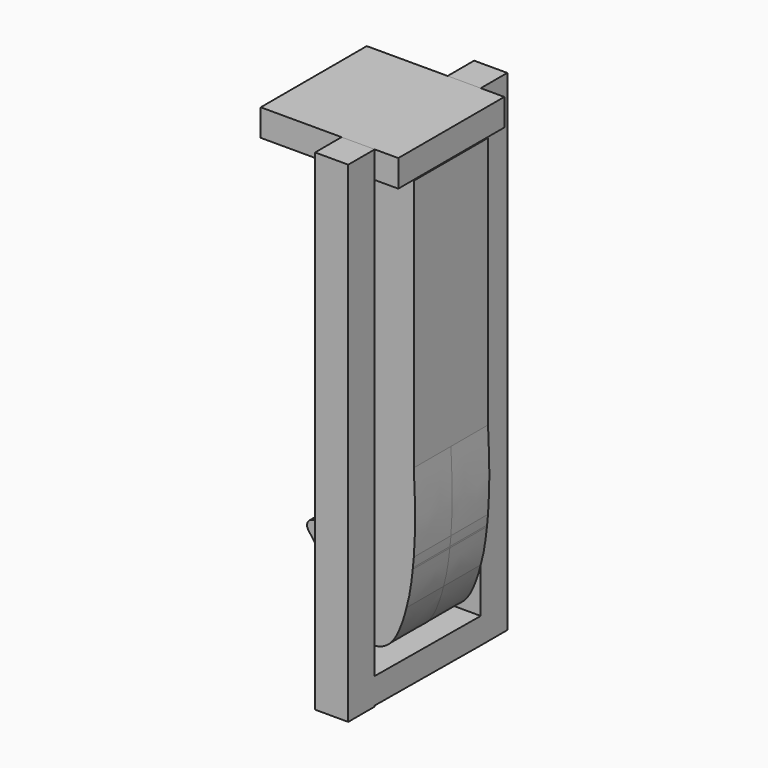
from build123d import *

# Parameters (mm, degrees)
F1_DEPTH = 8.89
F2_R     = 1.27
F3_R     = 1.27
F4_W     = 26.3627418317
F4_H     = 5.1619373262
F5_DEPTH = 12.7
F7_DEPTH = 6.35


with BuildPart() as f1:
    # F0 (on Front) → F1 (new body, symmetric)
    with BuildSketch(Plane.XZ):
        with BuildLine():
            add(Edge.make_bspline(
                [(4.2661379753, -33.616950048), (4.3349248687, -32.99222106), (4.3945578489, -32.36840068), (4.445, -31.75)],
                knots=[0.4799922653, 0.4799922653, 0.4799922653, 0.4799922653, 0.5123717025, 0.5123717025, 0.5123717025, 0.5123717025], degree=3))
            Line((4.445, -31.75), (-4.445, -31.75))
            Line((-4.445, -31.75), (-17.2371771187, -31.75))
            Line((-17.2371771187, -31.75), (-4.445, -49.3149235845))
            add(Edge.make_bspline(
                [(-4.445, -49.3149235845), (-2.8737867331, -49.1791167069), (-1.3025734662, -49.0433098293), (0, -47.6557277143)],
                knots=[0, 0, 0, 0, 0.1787943452, 0.1787943452, 0.1787943452, 0.1787943452], degree=3))
            add(Edge.make_bspline(
                [(0, -47.6557277143), (1.1546532493, -45.3808190167), (2.3218615323, -43.1096212641), (3.0350551164, -40.743494961)],
                knots=[0, 0, 0, 0, 0.5053639981, 0.5053639981, 0.5053639981, 0.5053639981], degree=3))
            add(Edge.make_bspline(
                [(3.0350551164, -40.743494961), (3.5641678247, -38.6195342287), (3.9647615791, -36.2559041312), (4.2348473132, -33.8956672077)],
                knots=[0.3528810834, 0.3528810834, 0.3528810834, 0.3528810834, 0.4751777864, 0.4751777864, 0.4751777864, 0.4751777864], degree=3))
            add(Edge.make_bspline(
                [(4.2348473132, -33.8956672077), (4.2452843652, -33.8027605788), (4.2557060854, -33.7098530506), (4.2661379753, -33.616950048)],
                knots=[0.9808831842, 0.9808831842, 0.9808831842, 0.9808831842, 1, 1, 1, 1], degree=3))
        make_face()
        with BuildLine():
            Line((-4.445, -31.75), (4.445, -31.75))
            Line((4.445, -31.75), (4.445, -16.6841130704))
            add(Edge.make_bspline(
                [(4.445, -16.6841130704), (4.390455432, -14.8693285963), (4.417727716, -13.6566404294), (4.445, -12.4439522624)],
                knots=[0.830976746, 0.830976746, 0.830976746, 0.830976746, 1, 1, 1, 1], degree=3))
            Line((4.445, -12.4439522624), (4.445, 31.75))
            Line((4.445, 31.75), (-4.445, 31.75))
            Line((-4.445, 31.75), (-4.445, -31.75))
        make_face()
        with BuildLine():
            Line((4.445, -16.6841130704), (4.445, -31.75))
            add(Edge.make_bspline(
                [(4.445, -31.75), (4.9413373419, -25.665101898), (4.5478152875, -20.1049411089), (4.445, -16.6841130704)],
                knots=[0.5123717025, 0.5123717025, 0.5123717025, 0.5123717025, 0.830976746, 0.830976746, 0.830976746, 0.830976746], degree=3))
        make_face()
        with BuildLine():
            add(Edge.make_bspline(
                [(4.445, -16.6841130704), (4.390455432, -14.8693285963), (4.417727716, -13.6566404294), (4.445, -12.4439522624)],
                knots=[0.830976746, 0.830976746, 0.830976746, 0.830976746, 1, 1, 1, 1], degree=3))
            Line((4.445, -16.6841130704), (4.445, -12.4439522624))
        make_face()
        with BuildLine():
            add(Edge.make_bspline(
                [(4.2348473132, -33.8956672077), (4.2454798326, -33.802751286), (4.2559100938, -33.709840623), (4.2661379753, -33.616950048)],
                knots=[0.4751777864, 0.4751777864, 0.4751777864, 0.4751777864, 0.4799922653, 0.4799922653, 0.4799922653, 0.4799922653], degree=3))
            add(Edge.make_bspline(
                [(4.2348473132, -33.8956672077), (4.2452843652, -33.8027605788), (4.2557060854, -33.7098530506), (4.2661379753, -33.616950048)],
                knots=[0.9808831842, 0.9808831842, 0.9808831842, 0.9808831842, 1, 1, 1, 1], degree=3))
        make_face()
        with BuildLine():
            add(Edge.make_bspline(
                [(3.0350551164, -40.743494961), (3.7061302896, -38.5171027806), (3.9752319818, -36.2066631893), (4.2348473132, -33.8956672077)],
                knots=[0.5053639981, 0.5053639981, 0.5053639981, 0.5053639981, 0.9808831842, 0.9808831842, 0.9808831842, 0.9808831842], degree=3))
            add(Edge.make_bspline(
                [(3.0350551164, -40.743494961), (3.5641678247, -38.6195342287), (3.9647615791, -36.2559041312), (4.2348473132, -33.8956672077)],
                knots=[0.3528810834, 0.3528810834, 0.3528810834, 0.3528810834, 0.4751777864, 0.4751777864, 0.4751777864, 0.4751777864], degree=3))
        make_face()
        with BuildLine():
            add(Edge.make_bspline(
                [(0, -47.6557277143), (1.2682770572, -46.3046802631), (2.2818745053, -43.7669075859), (3.0350551164, -40.743494961)],
                knots=[0.1787943452, 0.1787943452, 0.1787943452, 0.1787943452, 0.3528810834, 0.3528810834, 0.3528810834, 0.3528810834], degree=3))
            add(Edge.make_bspline(
                [(0, -47.6557277143), (1.1546532493, -45.3808190167), (2.3218615323, -43.1096212641), (3.0350551164, -40.743494961)],
                knots=[0, 0, 0, 0, 0.5053639981, 0.5053639981, 0.5053639981, 0.5053639981], degree=3))
        make_face()
    extrude(amount=F1_DEPTH, both=True)

    # F2
    f2_edges = [f1.edges().sort_by_distance(p)[0] for p in [
        (-17.237177, 0, -31.75),
    ]]
    fillet(f2_edges, radius=F2_R)

    # F3
    f3_edges = [f1.edges().sort_by_distance(p)[0] for p in [
        (-4.445, 4.445, -49.314924),
        (-4.445, -4.445, -49.314924),
    ]]
    fillet(f3_edges, radius=F3_R)


with BuildPart() as f5:
    # F4 (on Front) → F5 (new body, symmetric)
    with BuildSketch(Plane.XZ):
        with Locations((-8.6646776181, 34.5665309578)):
            Rectangle(F4_W, F4_H)
    extrude(amount=F5_DEPTH, both=True)


with BuildPart() as f7:
    # F6 (on Right) → F7 (new body)
    with BuildSketch(Plane.YZ):
        Polygon((19.05, 37.1474996209), (12.7, 37.1474996209), (12.7, -51.8958903849), (12.7, -56.8734705448), (19.05, -56.8734705448), align=None)
        Polygon((12.7, -56.8734705448), (12.7, -51.8958903849), (-12.7, -51.7115332186), (-12.7, -56.6891133785), align=None)
        Polygon((-12.7, -56.6891133785), (-12.7, -51.7115332186), (-12.7, 37.1474996209), (-19.05, 37.1474996209), (-19.05, -56.8734705448), (-12.7, -56.8734705448), align=None)
    extrude(amount=-F7_DEPTH)


solid = Compound([f1.part, f5.part, f7.part])
